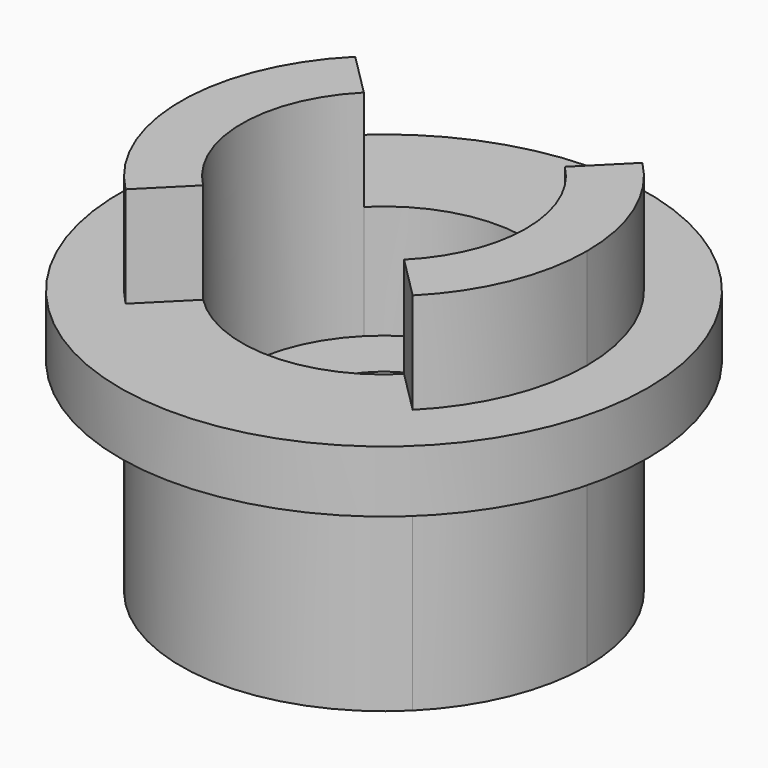
from build123d import *

# Parameters (mm, degrees)
F1_DEPTH = 63.5
F0_R     = 82.55
F2_DEPTH = 19.304
F3_DEPTH = 50.8
F4_DEPTH = 16.256


with BuildPart() as f1:
    # F0 (on Top) → F1 (new body)
    with BuildSketch(Plane.XY):
        with BuildLine():
            Line((-17.960512, 17.960512), (-31.430896, 31.430896))
            ThreePointArc((-31.430896, 31.430896), (-44.45, 0), (-31.430896, -31.430896))
            Line((-31.430896, -31.430896), (-17.960512, -17.960512))
            ThreePointArc((-17.960512, -17.960512), (-21.650197, -13.282656), (-24.148709, -7.874))
            Line((-24.148709, -7.874), (-32.022709, -7.874))
            Line((-32.022709, -7.874), (-32.022709, 7.874))
            Line((-32.022709, 7.874), (-24.148709, 7.874))
            ThreePointArc((-24.148709, 7.874), (-21.650197, 13.282656), (-17.960512, 17.960512))
        make_face()
        with BuildLine():
            Line((-31.430896, 31.430896), (-44.901281, 44.901281))
            ThreePointArc((-44.901281, 44.901281), (-63.5, 0), (-44.901281, -44.901281))
            Line((-44.901281, -44.901281), (-31.430896, -31.430896))
            ThreePointArc((-31.430896, -31.430896), (-44.45, 0), (-31.430896, 31.430896))
        make_face()
        with BuildLine():
            Line((31.430896, 31.430896), (44.901281, 44.901281))
            ThreePointArc((44.901281, 44.901281), (0, 63.5), (-44.901281, 44.901281))
            Line((-44.901281, 44.901281), (-31.430896, 31.430896))
            ThreePointArc((-31.430896, 31.430896), (0, 44.45), (31.430896, 31.430896))
        make_face()
        with BuildLine():
            Line((17.960512, 17.960512), (31.430896, 31.430896))
            ThreePointArc((31.430896, 31.430896), (0, 44.45), (-31.430896, 31.430896))
            Line((-31.430896, 31.430896), (-17.960512, 17.960512))
            ThreePointArc((-17.960512, 17.960512), (0, 25.4), (17.960512, 17.960512))
        make_face()
        with BuildLine():
            ThreePointArc((-31.430896, -31.430896), (0, -44.45), (31.430896, -31.430896))
            Line((31.430896, -31.430896), (17.960512, -17.960512))
            ThreePointArc((17.960512, -17.960512), (0, -25.4), (-17.960512, -17.960512))
            Line((-17.960512, -17.960512), (-31.430896, -31.430896))
        make_face()
        with BuildLine():
            ThreePointArc((-44.901281, -44.901281), (0, -63.5), (44.901281, -44.901281))
            Line((44.901281, -44.901281), (31.430896, -31.430896))
            ThreePointArc((31.430896, -31.430896), (0, -44.45), (-31.430896, -31.430896))
            Line((-31.430896, -31.430896), (-44.901281, -44.901281))
        make_face()
        with BuildLine():
            ThreePointArc((44.45, 0), (41.066445, 17.010279), (31.430896, 31.430896))
            Line((31.430896, 31.430896), (17.960512, 17.960512))
            ThreePointArc((17.960512, 17.960512), (23.46654, 9.720159), (25.4, 0))
            ThreePointArc((25.4, 0), (23.46654, -9.720159), (17.960512, -17.960512))
            Line((17.960512, -17.960512), (31.430896, -31.430896))
            ThreePointArc((31.430896, -31.430896), (41.066445, -17.010279), (44.45, 0))
        make_face()
        with BuildLine():
            ThreePointArc((44.901281, -44.901281), (58.66635, -24.300398), (63.5, 0))
            ThreePointArc((63.5, 0), (58.66635, 24.300398), (44.901281, 44.901281))
            Line((44.901281, 44.901281), (31.430896, 31.430896))
            ThreePointArc((31.430896, 31.430896), (41.066445, 17.010279), (44.45, 0))
            ThreePointArc((44.45, 0), (41.066445, -17.010279), (31.430896, -31.430896))
            Line((31.430896, -31.430896), (44.901281, -44.901281))
        make_face()
    extrude(amount=-F1_DEPTH)

    # F0 (on Top) → F2 (join)
    with BuildSketch(Plane.XY):
        Circle(F0_R)
        with BuildLine():
            ThreePointArc((44.901281, 44.901281), (58.66635, 24.300398), (63.5, 0))
            ThreePointArc((63.5, 0), (58.66635, -24.300398), (44.901281, -44.901281))
            ThreePointArc((44.901281, -44.901281), (0, -63.5), (-44.901281, -44.901281))
            ThreePointArc((-44.901281, -44.901281), (-63.5, 0), (-44.901281, 44.901281))
            ThreePointArc((-44.901281, 44.901281), (0, 63.5), (44.901281, 44.901281))
        make_face(mode=Mode.SUBTRACT)
        with BuildLine():
            Line((-31.430896, 31.430896), (-44.901281, 44.901281))
            ThreePointArc((-44.901281, 44.901281), (-63.5, 0), (-44.901281, -44.901281))
            Line((-44.901281, -44.901281), (-31.430896, -31.430896))
            ThreePointArc((-31.430896, -31.430896), (-44.45, 0), (-31.430896, 31.430896))
        make_face()
        with BuildLine():
            Line((31.430896, 31.430896), (44.901281, 44.901281))
            ThreePointArc((44.901281, 44.901281), (0, 63.5), (-44.901281, 44.901281))
            Line((-44.901281, 44.901281), (-31.430896, 31.430896))
            ThreePointArc((-31.430896, 31.430896), (0, 44.45), (31.430896, 31.430896))
        make_face()
        with BuildLine():
            ThreePointArc((-44.901281, -44.901281), (0, -63.5), (44.901281, -44.901281))
            Line((44.901281, -44.901281), (31.430896, -31.430896))
            ThreePointArc((31.430896, -31.430896), (0, -44.45), (-31.430896, -31.430896))
            Line((-31.430896, -31.430896), (-44.901281, -44.901281))
        make_face()
        with BuildLine():
            ThreePointArc((44.901281, -44.901281), (58.66635, -24.300398), (63.5, 0))
            ThreePointArc((63.5, 0), (58.66635, 24.300398), (44.901281, 44.901281))
            Line((44.901281, 44.901281), (31.430896, 31.430896))
            ThreePointArc((31.430896, 31.430896), (41.066445, 17.010279), (44.45, 0))
            ThreePointArc((44.45, 0), (41.066445, -17.010279), (31.430896, -31.430896))
            Line((31.430896, -31.430896), (44.901281, -44.901281))
        make_face()
    extrude(amount=F2_DEPTH)

    # F0 (on Top) → F3 (join)
    with BuildSketch(Plane.XY):
        with BuildLine():
            Line((-31.430896, 31.430896), (-44.901281, 44.901281))
            ThreePointArc((-44.901281, 44.901281), (-63.5, 0), (-44.901281, -44.901281))
            Line((-44.901281, -44.901281), (-31.430896, -31.430896))
            ThreePointArc((-31.430896, -31.430896), (-44.45, 0), (-31.430896, 31.430896))
        make_face()
        with BuildLine():
            ThreePointArc((44.901281, -44.901281), (58.66635, -24.300398), (63.5, 0))
            ThreePointArc((63.5, 0), (58.66635, 24.300398), (44.901281, 44.901281))
            Line((44.901281, 44.901281), (31.430896, 31.430896))
            ThreePointArc((31.430896, 31.430896), (41.066445, 17.010279), (44.45, 0))
            ThreePointArc((44.45, 0), (41.066445, -17.010279), (31.430896, -31.430896))
            Line((31.430896, -31.430896), (44.901281, -44.901281))
        make_face()
    extrude(amount=F3_DEPTH)

    # F4 (cut): a face of the model
    f4_faces = [f1.faces().sort_by_distance(p)[0] for p in [
        (-30.541896, -30.541896, 0),
    ]]
    extrude(f4_faces, amount=-F4_DEPTH, mode=Mode.SUBTRACT)


solid = f1.part
